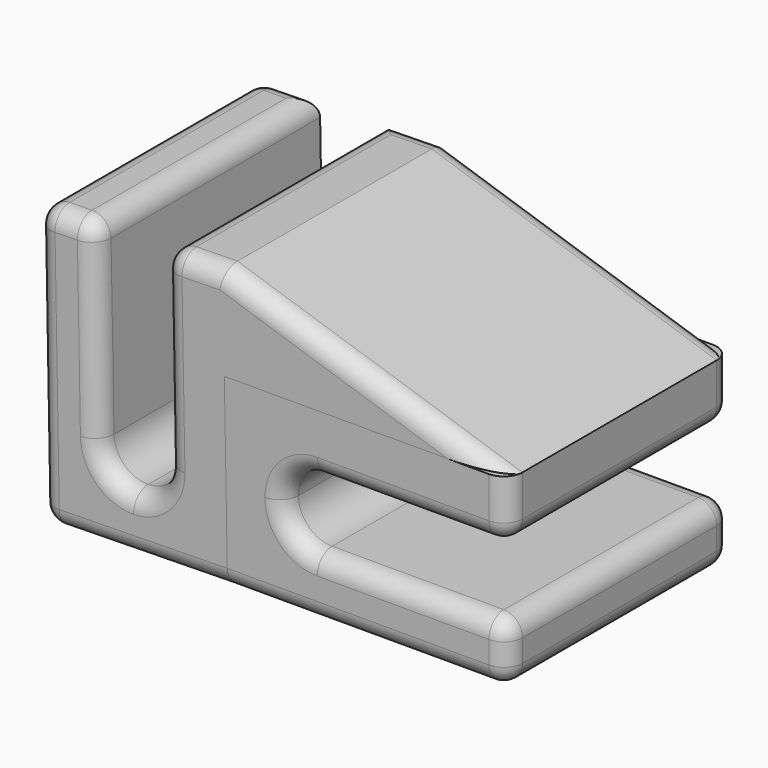
from build123d import *

# Parameters (mm, degrees)
F0_W     = 15
F0_H     = 15
F1_DEPTH = 10
F2_W     = 15
F2_H     = 3.6
F3_DEPTH = 12
F4_R     = 1.79999
F5_COUNT = 2
F5_ANGLE = 91
F7_DEPTH = 15
F9_DEPTH = 15
F10_R    = 1
F10_2_R  = 1


# Not quite as in the source:
# - a fillet or chamfer is up to 0.001 mm smaller than in the source, because OpenCascade refuses the exact size


with BuildPart() as f1:
    # F0 (on Top) → F1 (new body)
    with BuildSketch(Plane.XY):
        with Locations((7.5, 7.5)):
            Rectangle(F0_W, F0_H)
    extrude(amount=F1_DEPTH)

    # F2 (on face) → F3 (cut)
    with BuildSketch(Plane.YZ.offset(15)):
        with Locations((7.5, 5)):
            Rectangle(F2_W, F2_H)
    extrude(amount=-F3_DEPTH, mode=Mode.SUBTRACT)

    # F4 (radius 1.8 in the source; OpenCascade refuses exactly that, so slightly less here)
    f4_edges = [f1.edges().sort_by_distance(p)[0] for p in [
        (3, 7.5, 3.2),
        (3, 7.5, 6.8),
    ]]
    fillet(f4_edges, radius=F4_R)


with BuildPart() as f5_1:
    # F5: instance of F1
    add(f1.part.rotate(Axis((0, 7.5, 0), (0, -1, 0)), 1 * F5_ANGLE / (F5_COUNT - 1)))

    # F8 (on Front) → F9 (join, through all)
    with BuildSketch(Plane.XZ):
        Polygon((-0.2617860966, 14.9977154273), (-0.1745506493, 10), (15, 10), align=None)
    extrude(amount=-F9_DEPTH)

    # F10#2
    f10_2_edges = [f5_1.edges().sort_by_distance(p)[0] for p in [
        (-10.12937, 0, 7.324334),
        (-6.971743, 0, 9.779811),
        (-8.660507, 0, 14.851115),
        (-7.06075, 7.5, 14.879039),
        (-8.660507, 15, 14.851115),
        (-10.260263, 7.5, 14.823191),
        (-9.998477, 7.5, -0.174524),
        (-10.12937, 15, 7.324334),
        (-3.461299, 7.5, 14.941868),
        (-4.999238, 0, -0.087262),
        (-4.999238, 15, -0.087262),
        (-1.861542, 0, 14.969792),
        (7.369107, 0, 12.498858),
        (-1.861542, 15, 14.969792),
        (7.369107, 15, 12.498858),
        (-6.333398, 0, 3.417192),
        (-5.051596, 0, 2.912281),
        (-3.788195, 0, 3.461619),
        (-3.372291, 0, 9.842639),
    ]]
    fillet(f10_2_edges, radius=F10_2_R)


with BuildPart() as f1_1:
    add(f1.part)

    # F6 (on face) → F7 (join, through all)
    with BuildSketch(Plane.XZ):
        Polygon((0, 0), (0, 10), (-0.1745506493, 10), align=None)
    extrude(amount=-F7_DEPTH)

    # F10
    f10_edges = [f1_1.edges().sort_by_distance(p)[0] for p in [
        (9.899995, 0, 6.8),
        (15, 7.5, 6.8),
        (15, 15, 1.6),
        (15, 0, 1.6),
        (15, 7.5, 3.2),
        (9.899995, 15, 3.2),
        (15, 7.5, 0),
        (7.5, 0, 0),
        (7.5, 15, 0),
        (15, 0, 8.4),
        (15, 15, 8.4),
        (9.899995, 15, 6.8),
        (3.527205, 15, 3.727205),
        (3, 15, 5),
        (3.527205, 15, 6.272795),
        (3.527205, 0, 6.272795),
        (9.899995, 0, 3.2),
        (3, 0, 5),
        (3.527205, 0, 3.727205),
    ]]
    fillet(f10_edges, radius=F10_R)


solid = Compound([f5_1.part, f1_1.part])
